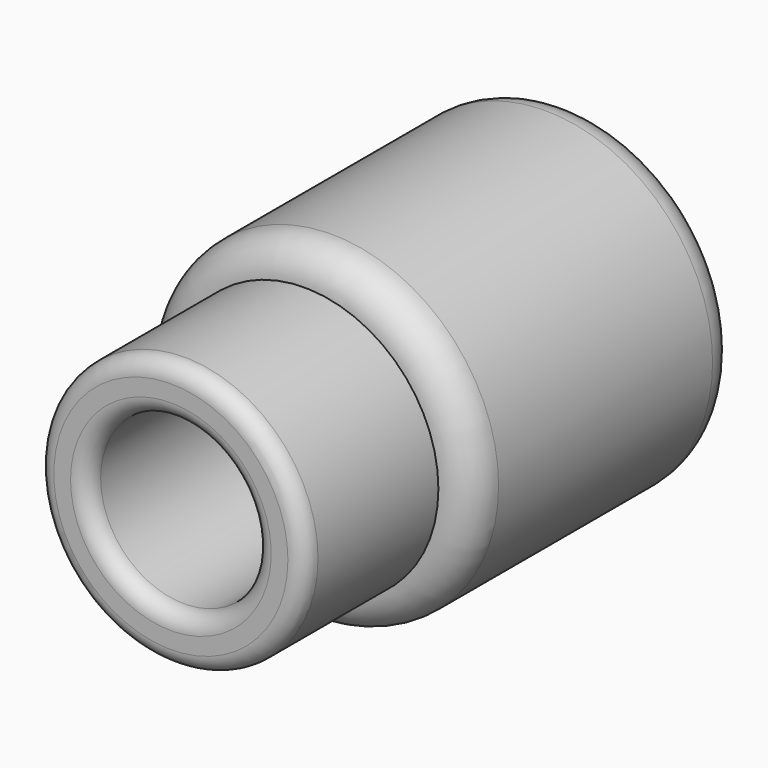
from build123d import *

# Parameters (mm, degrees)
F0_R     = 127
F1_DEPTH = 254
F2_R     = 25.4
F4_D     = 127
F5_DEPTH = 127
F6_R     = 12.7


# Not quite as in the source:
# - a feature names something its author has since deleted; it is built from what else it names


with BuildPart() as f1:
    # F0 (on Front) → F1 (new body)
    with BuildSketch(Plane.XZ):
        Circle(F0_R)
    extrude(amount=F1_DEPTH)

    # F2
    f2_edges = [f1.edges().sort_by_distance(p)[0] for p in [
        (-127, -254, 0),
        (-127, 0, 0),
    ]]
    fillet(f2_edges, radius=F2_R)

    # F4 (through all)
    with Locations(Plane.XZ.offset(254)):
        with Locations((0, 0)):
            Hole(F4_D / 2)

    # F5 (add): a face of the model
    f5_faces = [f1.faces().sort_by_distance(p)[0] for p in [
        (-98.7263180413, -254, 0),
    ]]
    extrude(f5_faces, amount=F5_DEPTH)

    # F6
    f6_edges = [f1.edges().sort_by_distance(p)[0] for p in [
        (-101.6, -381, 0),
        (-63.5, -381, 0),
    ]]
    fillet(f6_edges, radius=F6_R)


solid = f1.part
